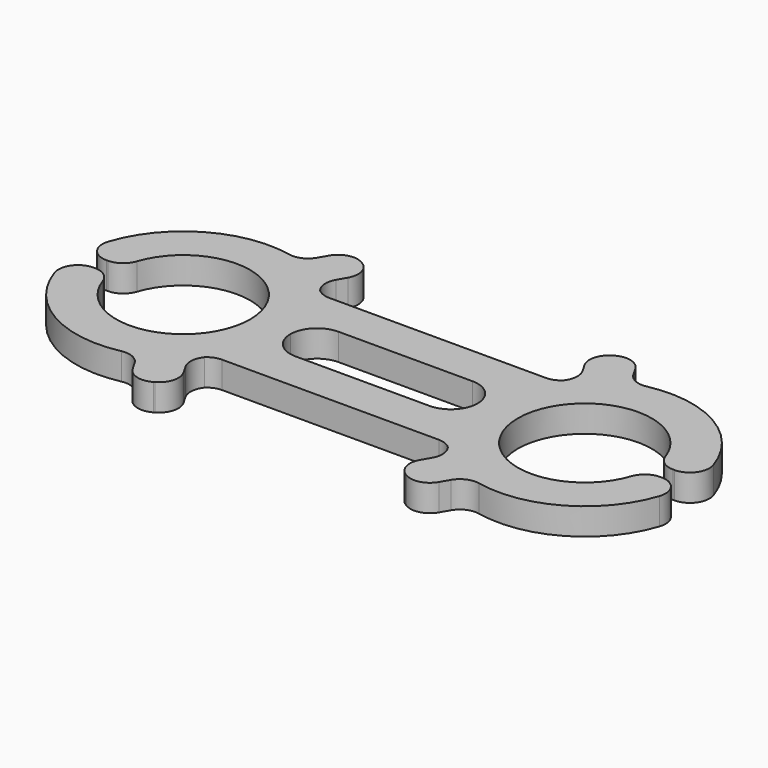
from build123d import *

# Parameters (mm, degrees)
F1_DEPTH     = 1.27
F2_R         = 6.35
F3_DEPTH     = 25.4
F4_W         = 12.6276115155
F4_H         = 1.524
F5_DEPTH     = 25.4
F7_DEPTH     = 25.4
F8_R         = 2.53999
F10_DEPTH    = 2.54
F11_T1_DEPTH = 2.54
F11_T3_DEPTH = 14.8669345535
F11_T5_DEPTH = 9.8531964618
F11_T7_DEPTH = 11.7475


# Not quite as in the source:
# - a fillet or chamfer that OpenCascade refuses, or shapes differently, is made with other operations: its cross-section is extruded or revolved along the edge and cut away or added
# - a fillet or chamfer is up to 0.001 mm smaller than in the source, because OpenCascade refuses the exact size


with BuildPart() as f1:
    # F0 (on Top) → F1 (new body, symmetric)
    with BuildSketch(Plane.XY):
        with BuildLine():
            ThreePointArc((-11.118852542, -6.35), (-9.4633932444, -3.3649028089), (-8.89, 0))
            ThreePointArc((-8.89, 0), (-9.4633932444, 3.3649028089), (-11.118852542, 6.35))
            ThreePointArc((-11.118852542, 6.35), (-29.21, 0), (-11.118852542, -6.35))
        make_face()
        with BuildLine():
            ThreePointArc((-11.118852542, 6.35), (-9.4633932444, 3.3649028089), (-8.89, 0))
            ThreePointArc((-8.89, 0), (-9.4633932444, -3.3649028089), (-11.118852542, -6.35))
            Line((-11.118852542, -6.35), (11.118852542, -6.35))
            ThreePointArc((11.118852542, -6.35), (8.89, 0), (11.118852542, 6.35))
            Line((11.118852542, 6.35), (-11.118852542, 6.35))
        make_face()
        with BuildLine():
            ThreePointArc((29.21, 0), (22.4149028089, 9.5866067556), (11.118852542, 6.35))
            ThreePointArc((11.118852542, 6.35), (8.89, 0), (11.118852542, -6.35))
            ThreePointArc((11.118852542, -6.35), (22.4149028089, -9.5866067556), (29.21, 0))
        make_face()
    extrude(amount=F1_DEPTH, both=True)

    # F2 (on face) → F3 (cut)
    with BuildSketch(Plane.XY.offset(1.27)):
        with Locations((-19.05, 0)):
            Circle(F2_R)
        with Locations((19.05, 0)):
            Circle(F2_R)
    extrude(amount=-F3_DEPTH, mode=Mode.SUBTRACT)

    # F4 (on face) → F5 (cut)
    with BuildSketch(Plane.XY.offset(1.27)):
        with Locations((-22.8961942422, 0)):
            Rectangle(F4_W, F4_H)
        with Locations((22.8961942422, 0)):
            Rectangle(F4_W, F4_H)
    extrude(amount=-F5_DEPTH, mode=Mode.SUBTRACT)

    # F6 (on face) → F7 (cut)
    with BuildSketch(Plane.XY.offset(1.27)):
        with BuildLine():
            ThreePointArc((-9.2126223006, 2.54), (-8.89, 0), (-9.2126223006, -2.54))
            Line((-9.2126223006, -2.54), (9.2126223006, -2.54))
            ThreePointArc((9.2126223006, -2.54), (8.89, 0), (9.2126223006, 2.54))
            Line((9.2126223006, 2.54), (-9.2126223006, 2.54))
        make_face()
    extrude(amount=-F7_DEPTH, mode=Mode.SUBTRACT)

    # F8 (radius 2.54 in the source; OpenCascade refuses exactly that, so slightly less here)
    f8_edges = [f1.edges().sort_by_distance(p)[0] for p in [
        (-9.212622, -2.54, 0),
        (-9.212622, 2.54, 0),
        (9.212622, 2.54, 0),
        (9.212622, -2.54, 0),
    ]]
    fillet(f8_edges, radius=F8_R)

    # F9 (on face) → F10 (join, through all)
    with BuildSketch(Plane.XY.offset(1.27)):
        Polygon((-13.6061572532, 13.2390122258), (-16.1461572532, 8.8396031746), (-12.8466004648, 6.9346031746), (-10.3066004648, 11.3340122258), align=None)
        Polygon((10.3066004648, 11.3340122258), (12.8466004648, 6.9346031746), (16.1461572532, 8.8396031746), (13.6061572532, 13.2390122258), align=None)
        Polygon((-12.8466004648, -6.9346031746), (-16.1461572532, -8.8396031746), (-13.6061572532, -13.2390122258), (-10.3066004648, -11.3340122258), align=None)
        Polygon((12.8466004648, -6.9346031746), (10.3066004648, -11.3340122258), (13.6061572532, -13.2390122258), (16.1461572532, -8.8396031746), align=None)
    extrude(amount=-F10_DEPTH)

    # F11: fillet of radius 1.8415 on 28 edges, made by hand

    # F11_s2 → F11_t1 (join)
    with BuildSketch(Plane.XY.offset(-1.27)):
        with BuildLine():
            ThreePointArc((-10.2787213019, -6.35), (-11.0123924632, -6.5024621446), (-11.6245788799, -6.9346031746))
            ThreePointArc((-11.6245788799, -6.9346031746), (-11.3661539682, -6.6471129191), (-11.118852542, -6.35))
            Line((-11.118852542, -6.35), (-10.2787213019, -6.35))
        make_face()
        with BuildLine():
            ThreePointArc((11.6245788799, -6.9346031746), (11.0123924632, -6.5024621446), (10.2787213019, -6.35))
            Line((10.2787213019, -6.35), (11.118852542, -6.35))
            ThreePointArc((11.118852542, -6.35), (11.3661539682, -6.6471129191), (11.6245788799, -6.9346031746))
        make_face()
        with BuildLine():
            ThreePointArc((11.6245788799, 6.9346031746), (11.0123924632, 6.5024621446), (10.2787213019, 6.35))
            Line((10.2787213019, 6.35), (11.118852542, 6.35))
            ThreePointArc((11.118852542, 6.35), (11.3661539682, 6.6471129191), (11.6245788799, 6.9346031746))
        make_face()
        with BuildLine():
            ThreePointArc((-11.6245788799, 6.9346031746), (-11.0123924632, 6.5024621446), (-10.2787213019, 6.35))
            Line((-10.2787213019, 6.35), (-11.118852542, 6.35))
            ThreePointArc((-11.118852542, 6.35), (-11.3661539682, 6.6471129191), (-11.6245788799, 6.9346031746))
        make_face()
        with BuildLine():
            ThreePointArc((-16.9705864556, 9.9449303321), (-15.8418987275, 10.0663992837), (-14.9989069696, 10.8266989549))
            Line((-14.9989069696, 10.8266989549), (-15.7098742118, 9.5952675689))
            ThreePointArc((-15.7098742118, 9.5952675689), (-16.3345962259, 9.790412777), (-16.9705864556, 9.9449303321))
        make_face()
        with BuildLine():
            ThreePointArc((-16.9705864556, -9.9449303321), (-15.8418987275, -10.0663992837), (-14.9989069696, -10.8266989549))
            Line((-14.9989069696, -10.8266989549), (-15.7098742118, -9.5952675689))
            ThreePointArc((-15.7098742118, -9.5952675689), (-16.3345962259, -9.790412777), (-16.9705864556, -9.9449303321))
        make_face()
        with BuildLine():
            ThreePointArc((-11.4771444657, -6.7732901205), (-11.9362931319, -7.8114968418), (-11.6993501812, -8.9216989549))
            Line((-11.6993501812, -8.9216989549), (-12.4103174233, -7.6902675689))
            ThreePointArc((-12.4103174233, -7.6902675689), (-11.9289557087, -7.2468150384), (-11.4771444657, -6.7732901205))
        make_face()
        with BuildLine():
            ThreePointArc((11.4771444657, -6.7732901205), (11.9362931319, -7.8114968418), (11.6993501812, -8.9216989549))
            Line((11.6993501812, -8.9216989549), (12.4103174233, -7.6902675689))
            ThreePointArc((12.4103174233, -7.6902675689), (11.9289557087, -7.2468150384), (11.4771444657, -6.7732901205))
        make_face()
        with BuildLine():
            ThreePointArc((16.9705864556, -9.9449303321), (15.8418987275, -10.0663992837), (14.9989069696, -10.8266989549))
            Line((14.9989069696, -10.8266989549), (15.7098742118, -9.5952675689))
            ThreePointArc((15.7098742118, -9.5952675689), (16.3345962259, -9.790412777), (16.9705864556, -9.9449303321))
        make_face()
        with BuildLine():
            ThreePointArc((11.4771444657, 6.7732901205), (11.9362931319, 7.8114968418), (11.6993501812, 8.9216989549))
            Line((11.6993501812, 8.9216989549), (12.4103174233, 7.6902675689))
            ThreePointArc((12.4103174233, 7.6902675689), (11.9289557087, 7.2468150384), (11.4771444657, 6.7732901205))
        make_face()
        with BuildLine():
            ThreePointArc((16.9705864556, 9.9449303321), (15.8418987275, 10.0663992837), (14.9989069696, 10.8266989549))
            Line((14.9989069696, 10.8266989549), (15.7098742118, 9.5952675689))
            ThreePointArc((15.7098742118, 9.5952675689), (16.3345962259, 9.790412777), (16.9705864556, 9.9449303321))
        make_face()
        with BuildLine():
            ThreePointArc((-11.4771444657, 6.7732901205), (-11.9362931319, 7.8114968418), (-11.6993501812, 8.9216989549))
            Line((-11.6993501812, 8.9216989549), (-12.4103174233, 7.6902675689))
            ThreePointArc((-12.4103174233, 7.6902675689), (-11.9289557087, 7.2468150384), (-11.4771444657, 6.7732901205))
        make_face()
    extrude(amount=F11_T1_DEPTH)

    # F11_s4 → F11_t3 (cut)
    with BuildSketch(Plane.XY.offset(-7.4334672767)):
        with BuildLine():
            ThreePointArc((-28.6995684343, 3.1798473282), (-28.4426407656, 1.5241996143), (-26.9505841556, 0.762))
            Line((-26.9505841556, 0.762), (-29.181384703, 0.762))
            ThreePointArc((-29.181384703, 0.762), (-29.0140866707, 1.9855923094), (-28.6995684343, 3.1798473282))
        make_face()
        with BuildLine():
            ThreePointArc((-26.9505841556, -0.762), (-28.4426407656, -1.5241996143), (-28.6995684343, -3.1798473282))
            ThreePointArc((-28.6995684343, -3.1798473282), (-29.0140866707, -1.9855923094), (-29.181384703, -0.762))
            Line((-29.181384703, -0.762), (-26.9505841556, -0.762))
        make_face()
        with BuildLine():
            ThreePointArc((26.9505841556, 0.762), (28.4426407656, 1.5241996143), (28.6995684343, 3.1798473282))
            ThreePointArc((28.6995684343, 3.1798473282), (29.0140866707, 1.9855923094), (29.181384703, 0.762))
            Line((29.181384703, 0.762), (26.9505841556, 0.762))
        make_face()
        with BuildLine():
            ThreePointArc((28.6995684343, -3.1798473282), (28.4426407656, -1.5241996143), (26.9505841556, -0.762))
            Line((26.9505841556, -0.762), (29.181384703, -0.762))
            ThreePointArc((29.181384703, -0.762), (29.0140866707, -1.9855923094), (28.6995684343, -3.1798473282))
        make_face()
    extrude(amount=F11_T3_DEPTH, mode=Mode.SUBTRACT)

    # F11_s6 → F11_t5 (cut)
    with BuildSketch(Plane.XY.offset(-4.9265982309)):
        with BuildLine():
            ThreePointArc((-26.8167535045, 0.762), (-25.7412713556, 1.1086888423), (-25.0707391508, 2.0182170543))
            ThreePointArc((-25.0707391508, 2.0182170543), (-25.244354117, 1.3973106575), (-25.3541142122, 0.762))
            Line((-25.3541142122, 0.762), (-26.8167535045, 0.762))
        make_face()
        with BuildLine():
            ThreePointArc((-25.0707391508, -2.0182170543), (-25.7412713556, -1.1086888423), (-26.8167535045, -0.762))
            Line((-26.8167535045, -0.762), (-25.3541142122, -0.762))
            ThreePointArc((-25.3541142122, -0.762), (-25.244354117, -1.3973106575), (-25.0707391508, -2.0182170543))
        make_face()
        with BuildLine():
            ThreePointArc((26.8167535045, -0.762), (25.7412713556, -1.1086888423), (25.0707391508, -2.0182170543))
            ThreePointArc((25.0707391508, -2.0182170543), (25.244354117, -1.3973106575), (25.3541142122, -0.762))
            Line((25.3541142122, -0.762), (26.8167535045, -0.762))
        make_face()
        with BuildLine():
            ThreePointArc((25.0707391508, 2.0182170543), (25.7412713556, 1.1086888423), (26.8167535045, 0.762))
            Line((26.8167535045, 0.762), (25.3541142122, 0.762))
            ThreePointArc((25.3541142122, 0.762), (25.244354117, 1.3973106575), (25.0707391508, 2.0182170543))
        make_face()
    extrude(amount=F11_T5_DEPTH, mode=Mode.SUBTRACT)

    # F11_s8 → F11_t7 (cut)
    with BuildSketch(Plane.XY.offset(-5.87375)):
        with BuildLine():
            ThreePointArc((-11.9013862459, -12.2547622258), (-11.0433838368, -11.1365917163), (-11.2273504648, -9.7392264448))
            Line((-11.2273504648, -9.7392264448), (-10.3066004648, -11.3340122258))
            Line((-10.3066004648, -11.3340122258), (-11.9013862459, -12.2547622258))
        make_face()
        with BuildLine():
            ThreePointArc((-14.5269072532, -11.6442264448), (-13.4087367437, -12.5022288539), (-12.0113714722, -12.3182622258))
            Line((-12.0113714722, -12.3182622258), (-13.6061572532, -13.2390122258))
            Line((-13.6061572532, -13.2390122258), (-14.5269072532, -11.6442264448))
        make_face()
        with BuildLine():
            ThreePointArc((11.2273504648, -9.7392264448), (11.0433838368, -11.1365917163), (11.9013862459, -12.2547622258))
            Line((11.9013862459, -12.2547622258), (10.3066004648, -11.3340122258))
            Line((10.3066004648, -11.3340122258), (11.2273504648, -9.7392264448))
        make_face()
        with BuildLine():
            ThreePointArc((12.0113714722, -12.3182622258), (13.4087367437, -12.5022288539), (14.5269072532, -11.6442264448))
            Line((14.5269072532, -11.6442264448), (13.6061572532, -13.2390122258))
            Line((13.6061572532, -13.2390122258), (12.0113714722, -12.3182622258))
        make_face()
        with BuildLine():
            ThreePointArc((14.5269072532, 11.6442264448), (13.4087367437, 12.5022288539), (12.0113714722, 12.3182622258))
            Line((12.0113714722, 12.3182622258), (13.6061572532, 13.2390122258))
            Line((13.6061572532, 13.2390122258), (14.5269072532, 11.6442264448))
        make_face()
        with BuildLine():
            ThreePointArc((11.9013862459, 12.2547622258), (11.0433838368, 11.1365917163), (11.2273504648, 9.7392264448))
            Line((11.2273504648, 9.7392264448), (10.3066004648, 11.3340122258))
            Line((10.3066004648, 11.3340122258), (11.9013862459, 12.2547622258))
        make_face()
        with BuildLine():
            ThreePointArc((-11.2273504648, 9.7392264448), (-11.0433838368, 11.1365917163), (-11.9013862459, 12.2547622258))
            Line((-11.9013862459, 12.2547622258), (-10.3066004648, 11.3340122258))
            Line((-10.3066004648, 11.3340122258), (-11.2273504648, 9.7392264448))
        make_face()
        with BuildLine():
            ThreePointArc((-12.0113714722, 12.3182622258), (-13.4087367437, 12.5022288539), (-14.5269072532, 11.6442264448))
            Line((-14.5269072532, 11.6442264448), (-13.6061572532, 13.2390122258))
            Line((-13.6061572532, 13.2390122258), (-12.0113714722, 12.3182622258))
        make_face()
    extrude(amount=F11_T7_DEPTH, mode=Mode.SUBTRACT)


solid = f1.part
